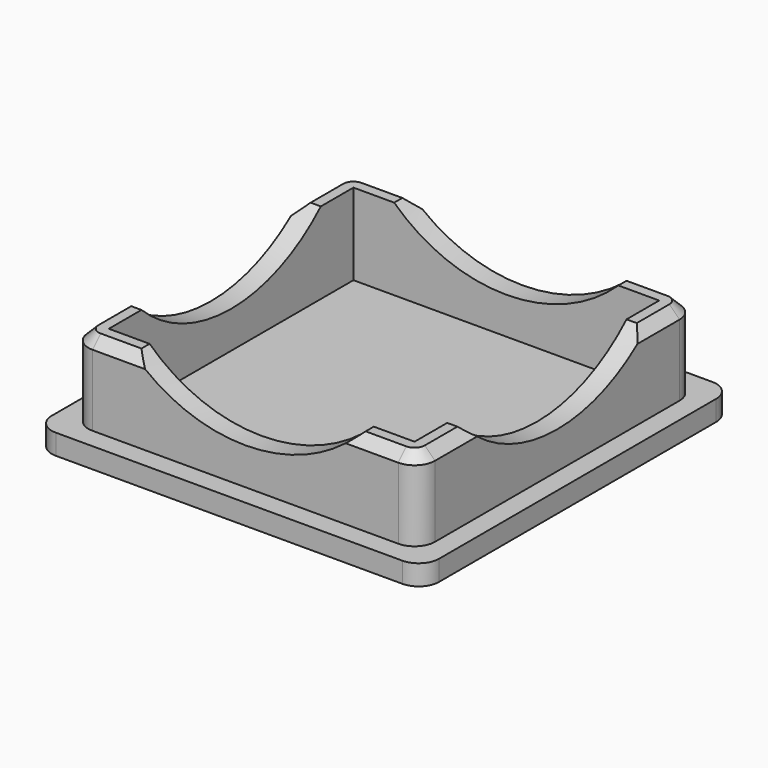
from build123d import *

# Parameters (mm, degrees)
F0_W            = 19
F0_H            = 19
F1_DEPTH        = 1
F2_W            = 17
F2_H            = 17
F3_DEPTH        = 4
F4_T            = 1
F4_T3_DEPTH     = 19
F4_T5_DEPTH     = 19
F6_DEPTH        = 2
F6_COPIES_COUNT = 4
F8_R            = 1
F9_SIZE         = 0.5


# Not quite as in the source:
# - a pattern or mirror of a feature is missing from the dataset's text; its kind, count and spacing are read off the source's solid
# - a shell that OpenCascade refuses in one call is made with other operations: the cavity is built on its own and cut out


with BuildPart() as f1:
    # F0 (on Top) → F1 (new body)
    with BuildSketch(Plane.XY):
        Rectangle(F0_W, F0_H)
    extrude(amount=F1_DEPTH)

    # F2 (on face) → F3 (join)
    with BuildSketch(Plane.XY.offset(1)):
        Rectangle(F2_W, F2_H)
    extrude(amount=F3_DEPTH)

    # F4: shell of thickness 1, made by hand


with BuildPart() as f4_core1:
    # F4_t2: copy of F1
    add(f1.part)

    # the walls: a layer under each face that stays
    f4_faces = [f4_core1.faces().sort_by_distance(p)[0] for p in [
        (0, -9.5, 0.5),
        (-9.5, 0, 0.5),
        (9.5, 0, 0.5),
        (0, 0, 0),
        (-8.8666666667, -8.8666666667, 1),
        (0, 9.5, 0.5),
        (8.5, 0, 3),
        (0, 8.5, 3),
        (-8.5, 0, 3),
        (0, -8.5, 3),
    ]]
    thicken(f4_faces, amount=-F4_T, mode=Mode.SUBTRACT)

    # F4_s4 → F4_t3 (cut)
    with BuildSketch(Plane.XZ.offset(-9.5)):
        Polygon((8.51, 1.01), (8.5, 0), (7.5, 0), (7.5, 1), align=None)
        Polygon((-8.51, 1.01), (-8.5, 0), (-7.5, 0), (-7.5, 1), align=None)
    extrude(amount=F4_T3_DEPTH, mode=Mode.SUBTRACT)

    # F4_s6 → F4_t5 (cut)
    with BuildSketch(Plane.YZ.offset(-9.5)):
        Polygon((8.51, 1.01), (8.5, 0), (7.5, 0), (7.5, 1), align=None)
        Polygon((-8.51, 1.01), (-8.5, 0), (-7.5, 0), (-7.5, 1), align=None)
    extrude(amount=F4_T5_DEPTH, mode=Mode.SUBTRACT)


with BuildPart() as f1_1:
    add(f1.part)

    # what is left inside the walls is the cavity
    f4_cavity = [f4_core1.part.solids().sort_by_distance(p)[0] for p in [
        (0, -2.5, 1.01),
    ]]
    add(f4_cavity, mode=Mode.SUBTRACT)

    # F5 (on face) → F6 (cut)
    with BuildSketch(Plane.XZ.offset(8.5)):
        with BuildLine():
            Line((5.5, 5), (-5.5, 5))
            ThreePointArc((-5.5, 5), (0, 2.8094750193), (5.5, 5))
        make_face()
    f6 = extrude(amount=-F6_DEPTH, mode=Mode.SUBTRACT)

    # F6_copies: F6 ×4 about axis
    f6_copies_axis = Axis((0, 0, 0), (0, 0, 1))
    for i in range(1, F6_COPIES_COUNT):
        add(f6.rotate(f6_copies_axis, i * 360 / F6_COPIES_COUNT), mode=Mode.SUBTRACT)

    # F8
    f8_edges = [f1_1.edges().sort_by_distance(p)[0] for p in [
        (-8.5, -8.5, 3),
        (-9.5, -9.5, 0.5),
        (8.5, -8.5, 3),
        (9.5, -9.5, 0.5),
        (8.5, 8.5, 3),
        (9.5, 9.5, 0.5),
        (-8.5, 8.5, 3),
        (-9.5, 9.5, 0.5),
    ]]
    fillet(f8_edges, radius=F8_R)

    # F9
    f9_edges = [f1_1.edges().sort_by_distance(p)[0] for p in [
        (6.5, 8.5, 5),
        (-6.5, 8.5, 5),
        (-8.5, 6.5, 5),
        (-8.5, -6.5, 5),
        (6.5, -8.5, 5),
        (8.5, -6.5, 5),
        (8.5, 6.5, 5),
        (8.207107, -8.207107, 5),
        (8.207107, 8.207107, 5),
        (-6.5, -8.5, 5),
        (-8.207107, -8.207107, 5),
        (-8.207107, 8.207107, 5),
    ]]
    chamfer(f9_edges, length=F9_SIZE)


solid = f1_1.part
